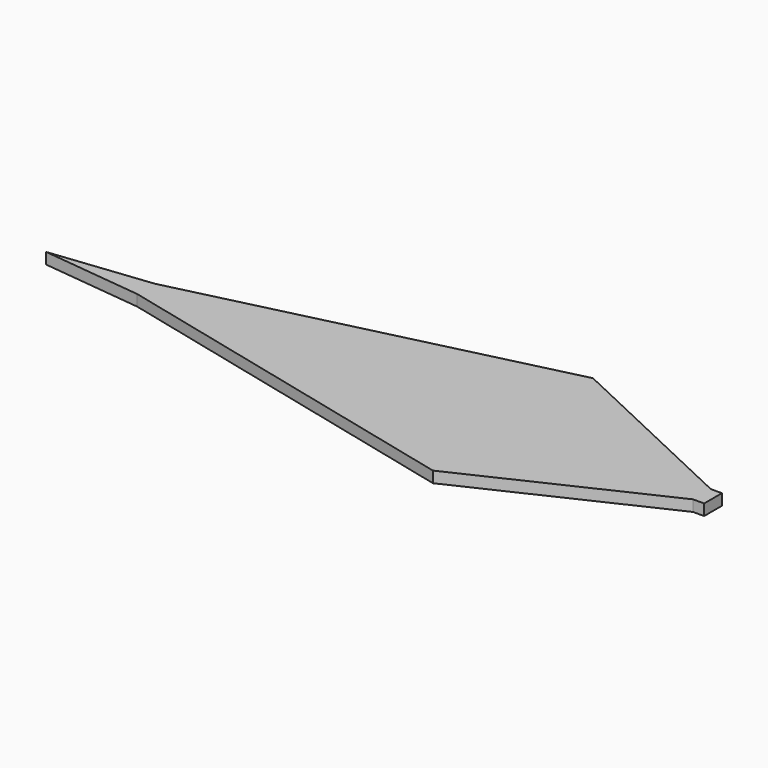
from build123d import *

# Parameters (mm, degrees)
F0_W     = 9.6744340956
F0_H     = 1
F1_DEPTH = 1


# Not quite as in the source:
# - a feature names something its author has since deleted; it is built from what else it names


with BuildPart() as f1:
    # F0 (on Top) → F1 (new body)
    with BuildSketch(Plane.XY):
        with Locations((-20.6627829522, 0.5)):
            Rectangle(F0_W, F0_H)
        Polygon((-34.5, 0), (-25.5, 0), (-25.5, 1), align=None)
        Polygon((-15.8255659044, 0), (-25.5, 0), (-25.5, -1), (24.5, -1), (25.5, -1), (25.5, 0), align=None)
        Polygon((-25.5, -1), (-25.5, 0), (-34.5, 0), align=None)
        Polygon((-15.8255659044, 1), (-15.8255659044, 0), (25.5, 0), (25.5, 1), (24.5, 1), align=None)
        with BuildLine():
            add(Edge.make_bspline(
                [(-25.5, 1), (-14.5003329962, 3.3801647369), (-13.2050132379, 2.5), (7.5, 3)],
                knots=[0, 0, 0, 0, 33.0605505096, 33.0605505096, 33.0605505096, 33.0605505096], degree=3))
            Line((-25.5, 1), (-15.8255659044, 1))
            Line((-15.8255659044, 1), (24.5, 1))
            add(Edge.make_bspline(
                [(7.5, 3), (14.1289979219, 2.5626332499), (18.8218969852, 1.9759975839), (24.5, 1)],
                knots=[0, 0, 0, 0, 17.1172427686, 17.1172427686, 17.1172427686, 17.1172427686], degree=3))
        make_face()
        with BuildLine():
            Line((7.5, 9), (-25.5, 1))
            add(Edge.make_bspline(
                [(-25.5, 1), (-14.5003329962, 3.3801647369), (-13.2050132379, 2.5), (7.5, 3)],
                knots=[0, 0, 0, 0, 33.0605505096, 33.0605505096, 33.0605505096, 33.0605505096], degree=3))
            add(Edge.make_bspline(
                [(7.5, 3), (14.1289979219, 2.5626332499), (18.8218969852, 1.9759975839), (24.5, 1)],
                knots=[0, 0, 0, 0, 17.1172427686, 17.1172427686, 17.1172427686, 17.1172427686], degree=3))
            Line((24.5, 1), (7.5, 9))
        make_face()
        with BuildLine():
            add(Edge.make_bspline(
                [(-25.5, -1), (-14.5003329962, -3.3801647369), (-13.2050132379, -2.5), (7.5, -3)],
                knots=[0, 0, 0, 0, 33.0605505096, 33.0605505096, 33.0605505096, 33.0605505096], degree=3))
            Line((-25.5, -1), (7.5, -9))
            Line((7.5, -9), (24.5, -1))
            add(Edge.make_bspline(
                [(7.5, -3), (14.1289979219, -2.5626332499), (18.8218969852, -1.9759975839), (24.5, -1)],
                knots=[0, 0, 0, 0, 17.1172427686, 17.1172427686, 17.1172427686, 17.1172427686], degree=3))
        make_face()
        with BuildLine():
            Line((24.5, -1), (-25.5, -1))
            add(Edge.make_bspline(
                [(-25.5, -1), (-14.5003329962, -3.3801647369), (-13.2050132379, -2.5), (7.5, -3)],
                knots=[0, 0, 0, 0, 33.0605505096, 33.0605505096, 33.0605505096, 33.0605505096], degree=3))
            add(Edge.make_bspline(
                [(7.5, -3), (14.1289979219, -2.5626332499), (18.8218969852, -1.9759975839), (24.5, -1)],
                knots=[0, 0, 0, 0, 17.1172427686, 17.1172427686, 17.1172427686, 17.1172427686], degree=3))
        make_face()
    extrude(amount=F1_DEPTH)


solid = f1.part
